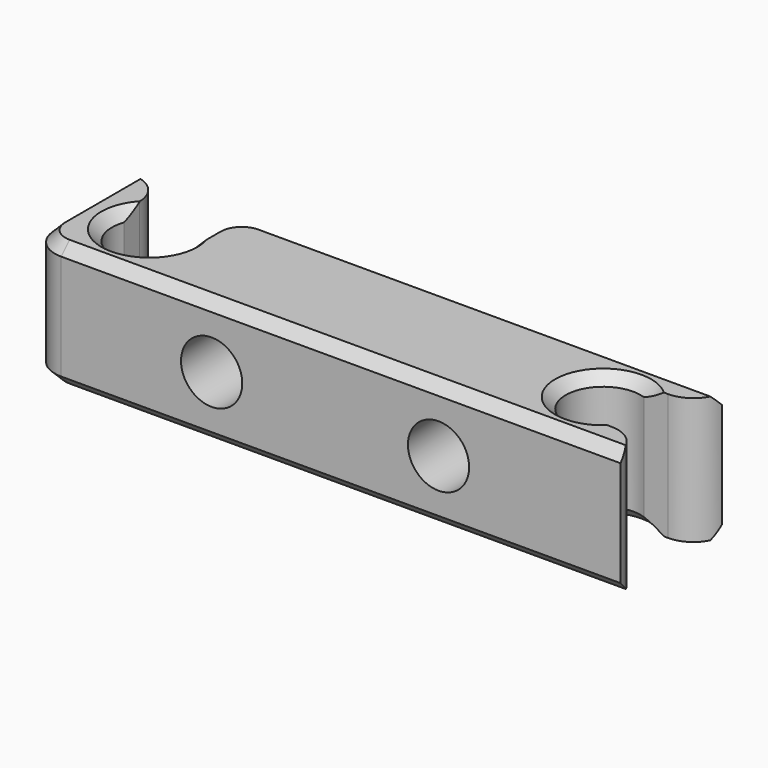
from build123d import *

# Parameters (mm, degrees)
F1_DEPTH    = 12
F3_T1_DEPTH = 27
F3_T3_DEPTH = 26.8975669154
F4_SIZE     = 1
F2_R        = 2.9
F5_DEPTH    = 12.001
F6_DEPTH    = 6


# Not quite as in the source:
# - a fillet or chamfer that OpenCascade refuses, or shapes differently, is made with other operations: its cross-section is extruded or revolved along the edge and cut away or added


with BuildPart() as f1:
    # F0 (on Top) → F1 (new body)
    with BuildSketch(Plane.XY):
        with BuildLine():
            Line((-24.8, 6), (-28, 6))
            Line((-28, 6), (-28, -6))
            Line((-28, -6), (28, -6))
            Line((28, -6), (28, -3.35))
            Line((28, -3.35), (22.7247340124, -3.35))
            ThreePointArc((22.7247340124, -3.35), (18, 0), (22.7247340124, 3.35))
            Line((22.7247340124, 3.35), (28, 3.35))
            Line((28, 3.35), (28, 6))
            Line((28, 6), (-18.1, 6))
            Line((-18.1, 6), (-18.1, 1.1747340124))
            ThreePointArc((-18.1, 1.1747340124), (-17.9503571611, 0.5958187644), (-17.9, 0))
            ThreePointArc((-17.9, 0), (-22.0458187644, -3.4996428389), (-24.8, 1.1747340124))
            Line((-24.8, 1.1747340124), (-24.8, 6))
        make_face()
    extrude(amount=F1_DEPTH)

    # F3: fillet of radius 3 on 5 edges, made by hand

    # F3_s2 → F3_t1 (cut)
    with BuildSketch(Plane.XY.offset(-7.5)):
        with BuildLine():
            ThreePointArc((-15.1, 6), (-17.2213203436, 5.1213203436), (-18.1, 3))
            Line((-18.1, 3), (-18.1, 6))
            Line((-18.1, 6), (-15.1, 6))
        make_face()
        with BuildLine():
            ThreePointArc((-27.8, 6), (-25.6786796564, 5.1213203436), (-24.8, 3))
            Line((-24.8, 3), (-24.8, 6))
            Line((-24.8, 6), (-27.8, 6))
        make_face()
        with BuildLine():
            ThreePointArc((-25, -6), (-27.1213203436, -5.1213203436), (-28, -3))
            Line((-28, -3), (-28, -6))
            Line((-28, -6), (-25, -6))
        make_face()
    extrude(amount=F3_T1_DEPTH, mode=Mode.SUBTRACT)

    # F3_s4 → F3_t3 (cut)
    with BuildSketch(Plane.XY.offset(-7.4487834577)):
        with BuildLine():
            ThreePointArc((25.0204866169, -3.35), (27.0142268206, -4.1083488229), (28, -6))
            Line((28, -6), (28, -3.35))
            Line((28, -3.35), (25.0204866169, -3.35))
        make_face()
        with BuildLine():
            ThreePointArc((28, 6), (27.0142268206, 4.1083488229), (25.0204866169, 3.35))
            Line((25.0204866169, 3.35), (28, 3.35))
            Line((28, 3.35), (28, 6))
        make_face()
    extrude(amount=F3_T3_DEPTH, mode=Mode.SUBTRACT)

    # F4
    f4_edges = [f1.edges().sort_by_distance(p)[0] for p in [
        (1.5, -6, 12),
        (1.5, -6, 0),
        (18, 0, 12),
        (-21.45, -3.55, 12),
        (18, 0, 0),
        (-21.45, -3.55, 0),
        (6.45, 6, 0),
        (6.45, 6, 12),
        (-18.1, 2.087367, 0),
        (-17.22132, 5.12132, 0),
        (-27.12132, -5.12132, 0),
        (-28, 1.5, 0),
        (-18.1, 2.087367, 12),
        (-17.22132, 5.12132, 12),
        (-27.12132, -5.12132, 12),
        (-28, 1.5, 12),
    ]]
    chamfer(f4_edges, length=F4_SIZE)

    # F2 (on face) → F5 (cut, through all)
    with BuildSketch(Plane(origin=(0, 6, 0), x_dir=(-1, 0, 0), z_dir=(0, 1, 0))):
        with Locations((-10.75, 6)):
            Circle(F2_R)
        with Locations((10.75, 6)):
            Circle(F2_R)
    extrude(amount=-F5_DEPTH, mode=Mode.SUBTRACT)

    # F2 (on face) → F6 (cut)
    with BuildSketch(Plane(origin=(0, 6, 0), x_dir=(-1, 0, 0), z_dir=(0, 1, 0))):
        Polygon((-7.8921161675, 10.95), (-13.6078838325, 10.95), (-16.465767665, 6), (-13.6078838325, 1.05), (-7.8921161675, 1.05), (-5.034232335, 6), align=None)
        with Locations((-10.75, 6)):
            Circle(F2_R, mode=Mode.SUBTRACT)
        Polygon((13.6078838325, 10.95), (7.8921161675, 10.95), (5.034232335, 6), (7.8921161675, 1.05), (13.6078838325, 1.05), (16.465767665, 6), align=None)
        with Locations((10.75, 6)):
            Circle(F2_R, mode=Mode.SUBTRACT)
    extrude(amount=-F6_DEPTH, mode=Mode.SUBTRACT)


solid = f1.part
